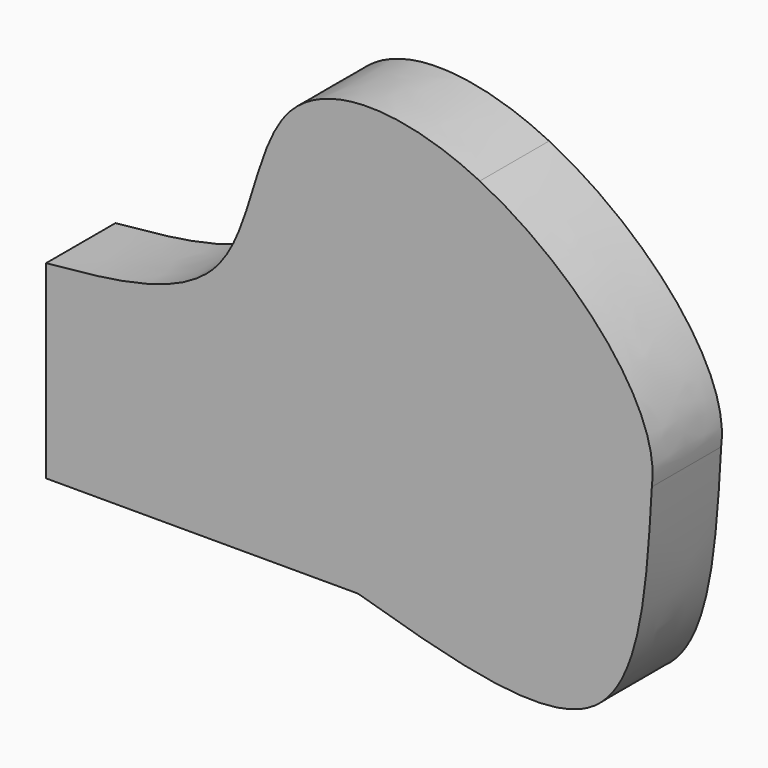
from build123d import *

# Parameters (mm, degrees)
F0_W     = 55.5266755181
F0_H     = 46.0978470142
F1_DEPTH = 25.4


with BuildPart() as f1:
    # F0 (on Front) → F1 (new body)
    with BuildSketch(Plane.XZ):
        Polygon((-45.72, 27.7720657421), (-45.72, -27.7720657421), (45.72, -27.7720657421), (45.72, 2.3720657421), (45.72, 27.7720657421), align=None)
        with BuildLine():
            Line((45.72, 2.3720657421), (45.72, -27.7720657421))
            add(Edge.make_bspline(
                [(131.83991611, 27.7720657421), (128.4226083131, 3.6394915706), (87.0713041565, -12.0662870858), (45.72, -27.7720657421)],
                knots=[0.7528337274, 0.7528337274, 0.7528337274, 0.7528337274, 1, 1, 1, 1], degree=3))
            add(Edge.make_bspline(
                [(81.4163490426, 90.3064464871), (108.1552290461, 77.110332117), (134.8655063082, 49.1383822136), (131.83991611, 27.7720657421)],
                knots=[0.5339995176, 0.5339995176, 0.5339995176, 0.5339995176, 0.7528337274, 0.7528337274, 0.7528337274, 0.7528337274], degree=3))
            Line((81.4163490426, 90.3064464871), (104.9052251901, 53.874658511))
            ThreePointArc((104.9052251901, 53.874658511), (101.4010974206, 18.9161297578), (70.4063948109, 2.3720657421))
            Line((70.4063948109, 2.3720657421), (45.72, 2.3720657421))
        make_face()
        with BuildLine():
            add(Edge.make_bspline(
                [(131.83991611, 27.7720657421), (128.4226083131, 3.6394915706), (87.0713041565, -12.0662870858), (45.72, -27.7720657421)],
                knots=[0.7528337274, 0.7528337274, 0.7528337274, 0.7528337274, 1, 1, 1, 1], degree=3))
            add(Edge.make_bspline(
                [(45.72, -27.7720657421), (73.2817283043, -35.9046962959), (100.8434566087, -44.0373268496), (115.1341721416, -34.0887419879)],
                knots=[0, 0, 0, 0, 0.5105148873, 0.5105148873, 0.5105148873, 0.5105148873], degree=3))
            add(Edge.make_bspline(
                [(115.1341721416, -34.0887419879), (128.8362064561, -24.5499718093), (130.3380612831, 1.6110469664), (131.83991611, 27.7720657421)],
                knots=[0.5105148873, 0.5105148873, 0.5105148873, 0.5105148873, 1, 1, 1, 1], degree=3))
        make_face()
        with BuildLine():
            add(Edge.make_bspline(
                [(-45.72, 27.7720657421), (-25.4090292575, 29.6505869851), (-5.0980585151, 31.5291082281), (5.0941300286, 44.2085994729)],
                knots=[0, 0, 0, 0, 0.1784307554, 0.1784307554, 0.1784307554, 0.1784307554], degree=3))
            Line((-45.72, 27.7720657421), (45.72, 27.7720657421))
            Line((45.72, 27.7720657421), (70.4063948109, 27.7720657421))
            ThreePointArc((70.4063948109, 27.7720657421), (80.2980419597, 33.0519371353), (81.4163490426, 44.2085994729))
            Line((81.4163490426, 44.2085994729), (25.8896735245, 44.2085994729))
            Line((25.8896735245, 44.2085994729), (5.0941300286, 44.2085994729))
        make_face()
        with BuildLine():
            Line((45.72, 27.7720657421), (45.72, 2.3720657421))
            Line((45.72, 2.3720657421), (70.4063948109, 2.3720657421))
            ThreePointArc((70.4063948109, 2.3720657421), (101.4010974206, 18.9161297578), (104.9052251901, 53.874658511))
            Line((104.9052251901, 53.874658511), (81.4163490426, 44.2085994729))
            ThreePointArc((81.4163490426, 44.2085994729), (80.2980419597, 33.0519371353), (70.4063948109, 27.7720657421))
            Line((70.4063948109, 27.7720657421), (45.72, 27.7720657421))
        make_face()
        with BuildLine():
            add(Edge.make_bspline(
                [(5.0941300286, 44.2085994729), (15.012118023, 56.5469742394), (15.3484515231, 79.1129792412), (25.8896735245, 90.3064464871)],
                knots=[0.1784307554, 0.1784307554, 0.1784307554, 0.1784307554, 0.3520611864, 0.3520611864, 0.3520611864, 0.3520611864], degree=3))
            Line((5.0941300286, 44.2085994729), (25.8896735245, 44.2085994729))
            Line((25.8896735245, 44.2085994729), (25.8896735245, 90.3064464871))
        make_face()
        with Locations((53.6530112836, 67.25752298)):
            Rectangle(F0_W, F0_H)
        Polygon((104.9052251901, 53.874658511), (81.4163490426, 90.3064464871), (81.4163490426, 44.2085994729), align=None)
        with BuildLine():
            Line((25.8896735245, 90.3064464871), (81.4163490426, 90.3064464871))
            add(Edge.make_bspline(
                [(25.8896735245, 90.3064464871), (36.9352738157, 102.0355007707), (59.185696861, 101.2776699891), (81.4163490426, 90.3064464871)],
                knots=[0.3520611864, 0.3520611864, 0.3520611864, 0.3520611864, 0.5339995176, 0.5339995176, 0.5339995176, 0.5339995176], degree=3))
        make_face()
    extrude(amount=F1_DEPTH)


solid = f1.part
